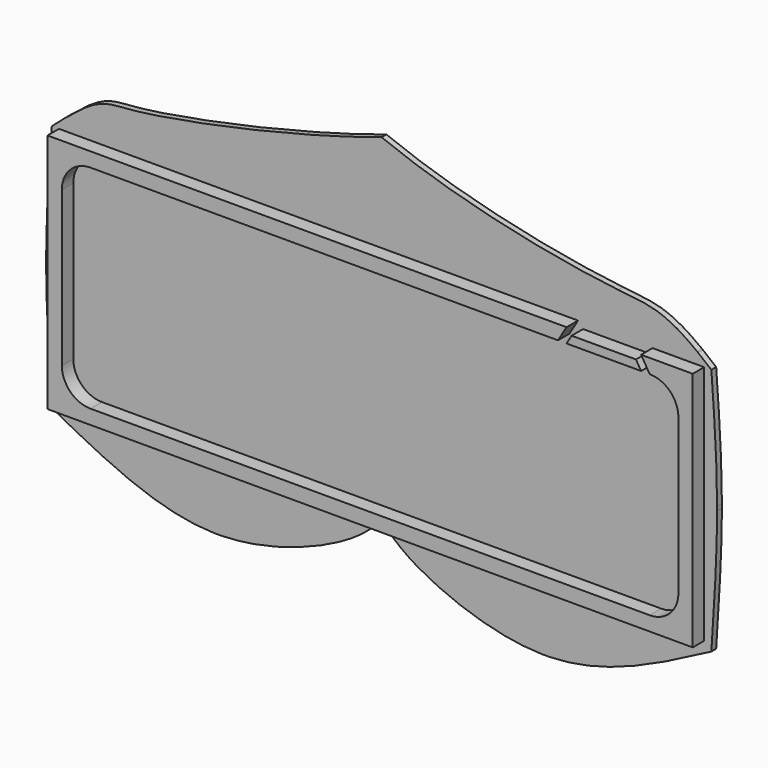
from build123d import *

# Parameters (mm, degrees)
F0_W     = 584.2
F0_H     = 219.71
F1_DEPTH = 5.334
F2_W     = 571.5
F2_H     = 213.36
F2_W_2   = 546.1
F2_H_2   = 187.96
F3_DEPTH = 12.7
F4_R     = 25.4
F6_DEPTH = 12.7
F8_DEPTH = 5.334
F9_DEPTH = 5.334


# Not quite as in the source:
# - a feature names something its author has since deleted; it is built from what else it names


with BuildPart() as f1:
    # F0 (on Front) → F1 (new body)
    with BuildSketch(Plane.XZ):
        with Locations((-292.1, 109.855)):
            Rectangle(F0_W, F0_H)
    extrude(amount=F1_DEPTH)

    # F2 (on face) → F3 (join)
    with BuildSketch(Plane.XZ.offset(5.334)):
        with Locations((-292.1, 113.03)):
            Rectangle(F2_W, F2_H)
        with Locations((-292.1, 113.03)):
            Rectangle(F2_W_2, F2_H_2, mode=Mode.SUBTRACT)
    extrude(amount=F3_DEPTH)

    # F4
    f4_edges = [f1.edges().sort_by_distance(p)[0] for p in [
        (-565.15, -11.684, 207.01),
        (-19.05, -11.684, 207.01),
        (-19.05, -11.684, 19.05),
        (-565.15, -11.684, 19.05),
    ]]
    fillet(f4_edges, radius=F4_R)

    # F5 (on face) → F6 (cut)
    with BuildSketch(Plane.XZ.offset(18.034)):
        Polygon((-118.11, 219.71), (-125.73, 207.01), (-118.11, 207.01), (-113.5820166854, 214.5566388576), (-110.49, 219.71), align=None)
        Polygon((-56.5979833146, 214.5566388576), (-52.07, 207.01), (-44.45, 207.01), (-52.07, 219.71), (-59.69, 219.71), align=None)
        Polygon((-59.69, 219.71), (-110.49, 219.71), (-113.5820166854, 214.5566388576), (-56.5979833146, 214.5566388576), align=None)
    extrude(amount=-F6_DEPTH, mode=Mode.SUBTRACT)

    # F7 (on face) → F8 (cut)
    with BuildSketch(Plane(origin=(0, 0, 0), x_dir=(-1, 0, 0), z_dir=(0, 1, 0))):
        with BuildLine():
            add(Edge.make_bspline(
                [(292.1, 6.35), (289.8878914708, 4.2388101088), (287.6757829415, 2.1276202176), (285.3383261504, 0)],
                knots=[0, 0, 0, 0, 0.0566650496, 0.0566650496, 0.0566650496, 0.0566650496], degree=3))
            Line((285.3383261504, 0), (292.1, 0))
            Line((292.1, 0), (292.1, 6.35))
        make_face()
        with BuildLine():
            add(Edge.make_bspline(
                [(292.1, 6.35), (294.3115112442, 4.2388053382), (296.5230224884, 2.1276106765), (298.8599853109, 0)],
                knots=[0, 0, 0, 0, 0.056662645, 0.056662645, 0.056662645, 0.056662645], degree=3))
            Line((292.1, 6.35), (292.1, 0))
            Line((292.1, 0), (298.8599853109, 0))
        make_face()
    extrude(amount=-F8_DEPTH, mode=Mode.SUBTRACT)

    # F7 (on face) → F9 (join)
    with BuildSketch(Plane(origin=(0, 0, 0), x_dir=(-1, 0, 0), z_dir=(0, 1, 0))):
        with BuildLine():
            Line((285.3383261504, 0), (0, 0))
            add(Edge.make_bspline(
                [(35.5548654074, -18.4164866805), (23.6750755263, -12.5314961521), (11.8375377632, -6.265748076), (0, 0)],
                knots=[0.8952858021, 0.8952858021, 0.8952858021, 0.8952858021, 1, 1, 1, 1], degree=3))
            Line((35.5548654074, -18.4164866805), (260.35, -18.4164866805))
            add(Edge.make_bspline(
                [(285.3383261504, 0), (278.8607301271, -5.8960937002), (271.4205053001, -11.9183662972), (260.35, -18.4164866805)],
                knots=[0.0566650496, 0.0566650496, 0.0566650496, 0.0566650496, 0.2136961022, 0.2136961022, 0.2136961022, 0.2136961022], degree=3))
        make_face()
        with BuildLine():
            add(Edge.make_bspline(
                [(0, 0), (-2.5016001756, 37.5778391816), (-5.0032003512, 75.1556783631), (-5.08, 111.5191693883)],
                knots=[0, 0, 0, 0, 0.4959951232, 0.4959951232, 0.4959951232, 0.4959951232], degree=3))
            Line((0, 0), (0, 219.71))
            add(Edge.make_bspline(
                [(-5.08, 114.935), (-5.0035853497, 150.6697582461), (-2.5017926748, 185.189879123), (0, 219.71)],
                knots=[0.5115421197, 0.5115421197, 0.5115421197, 0.5115421197, 1, 1, 1, 1], degree=3))
            Line((-5.08, 114.935), (-5.08, 111.5191693883))
        make_face()
        with BuildLine():
            Line((260.35, -18.4164866805), (35.5548654074, -18.4164866805))
            add(Edge.make_bspline(
                [(143.5928555626, -50.8), (106.470496214, -50.0055886792), (70.8264502644, -35.8892656507), (35.5548654074, -18.4164866805)],
                knots=[0.5843850409, 0.5843850409, 0.5843850409, 0.5843850409, 0.8952858021, 0.8952858021, 0.8952858021, 0.8952858021], degree=3))
            Line((143.5928555626, -50.8), (150.3785817486, -50.8))
            add(Edge.make_bspline(
                [(260.35, -18.4164866805), (235.5497171967, -32.973656279), (192.5306851802, -49.9188924594), (150.3785817486, -50.8)],
                knots=[0.2136961022, 0.2136961022, 0.2136961022, 0.2136961022, 0.5654790071, 0.5654790071, 0.5654790071, 0.5654790071], degree=3))
        make_face()
        with BuildLine():
            add(Edge.make_bspline(
                [(11.7731056729, 229.2938254471), (8.1151931686, 226.4637173569), (4.2088787391, 223.2851496368), (0, 219.71)],
                knots=[0.9578423111, 0.9578423111, 0.9578423111, 0.9578423111, 1, 1, 1, 1], degree=3))
            Line((0, 219.71), (292.1, 219.71))
            Line((292.1, 219.71), (11.7731056729, 229.2938254471))
        make_face()
        with BuildLine():
            add(Edge.make_bspline(
                [(12.5206463088, 229.87), (12.2726179558, 229.6795636028), (12.0234435309, 229.4875105602), (11.7731056729, 229.2938254471)],
                knots=[0.9549571504, 0.9549571504, 0.9549571504, 0.9549571504, 0.9578423111, 0.9578423111, 0.9578423111, 0.9578423111], degree=3))
            Line((11.7731056729, 229.2938254471), (292.1, 219.71))
            Line((292.1, 219.71), (573.1817260974, 229.3196316614))
            add(Edge.make_bspline(
                [(572.5320605941, 229.87), (572.7473841939, 229.6879525114), (572.9639346328, 229.5045002197), (573.1817260974, 229.3196316614)],
                knots=[0.9616983958, 0.9616983958, 0.9616983958, 0.9616983958, 0.9640299265, 0.9640299265, 0.9640299265, 0.9640299265], degree=3))
            Line((572.5320605941, 229.87), (514.35, 229.87))
            Line((514.35, 229.87), (292.1, 229.87))
            Line((292.1, 229.87), (82.55, 229.87))
            Line((82.55, 229.87), (12.5206463088, 229.87))
        make_face()
        with BuildLine():
            Line((573.1817260974, 229.3196316614), (292.1, 219.71))
            Line((292.1, 219.71), (584.2, 219.71))
            add(Edge.make_bspline(
                [(573.1817260974, 229.3196316614), (576.5417396252, 226.4675416698), (580.1971331881, 223.2783621084), (584.2, 219.71)],
                knots=[0.9640299265, 0.9640299265, 0.9640299265, 0.9640299265, 1, 1, 1, 1], degree=3))
        make_face()
        with BuildLine():
            add(Edge.make_bspline(
                [(298.8599853109, 0), (305.3364495341, -5.8962831133), (312.7764065366, -11.9186444461), (323.85, -18.4164866805)],
                knots=[0.056662645, 0.056662645, 0.056662645, 0.056662645, 0.2136927825, 0.2136927825, 0.2136927825, 0.2136927825], degree=3))
            Line((323.85, -18.4164866805), (548.6673215949, -18.4164866805))
            add(Edge.make_bspline(
                [(548.6673215949, -18.4164866805), (560.540064076, -12.5314899408), (572.370032038, -6.2657449704), (584.2, 0)],
                knots=[0.8952964295, 0.8952964295, 0.8952964295, 0.8952964295, 1, 1, 1, 1], degree=3))
            Line((584.2, 0), (298.8599853109, 0))
        make_face()
        with BuildLine():
            Line((548.6673215949, -18.4164866805), (323.85, -18.4164866805))
            add(Edge.make_bspline(
                [(323.85, -18.4164866805), (348.6543054028, -32.9713340996), (391.6899454814, -49.9118498543), (433.8458201185, -50.8)],
                knots=[0.2136927825, 0.2136927825, 0.2136927825, 0.2136927825, 0.5654325768, 0.5654325768, 0.5654325768, 0.5654325768], degree=3))
            Line((433.8458201185, -50.8), (440.69, -50.8))
            add(Edge.make_bspline(
                [(440.69, -50.8), (477.8051745876, -49.9992725657), (513.4246952416, -35.8853016167), (548.6673215949, -18.4164866805)],
                knots=[0.5844980763, 0.5844980763, 0.5844980763, 0.5844980763, 0.8952964295, 0.8952964295, 0.8952964295, 0.8952964295], degree=3))
        make_face()
        with BuildLine():
            add(Edge.make_bspline(
                [(82.55, 255.27), (55.6261452853, 252.2921647864), (42.3764019315, 252.7932765823), (12.5206463088, 229.87)],
                knots=[0.6076635734, 0.6076635734, 0.6076635734, 0.6076635734, 0.9549571504, 0.9549571504, 0.9549571504, 0.9549571504], degree=3))
            Line((12.5206463088, 229.87), (82.55, 229.87))
            Line((82.55, 229.87), (82.55, 255.27))
        make_face()
        with BuildLine():
            add(Edge.make_bspline(
                [(589.28, 114.935), (589.2035853497, 150.6697582461), (586.7017926748, 185.189879123), (584.2, 219.71)],
                knots=[0.5115421197, 0.5115421197, 0.5115421197, 0.5115421197, 1, 1, 1, 1], degree=3))
            Line((584.2, 219.71), (584.2, 0))
            add(Edge.make_bspline(
                [(584.2, 0), (586.7016001756, 37.5778391816), (589.2032003512, 75.1556783632), (589.28, 111.5191693884)],
                knots=[0, 0, 0, 0, 0.4959951232, 0.4959951232, 0.4959951232, 0.4959951232], degree=3))
            Line((589.28, 111.5191693884), (589.28, 114.935))
        make_face()
        with BuildLine():
            Line((82.55, 255.27), (82.55, 229.87))
            Line((82.55, 229.87), (292.1, 229.87))
            Line((292.1, 229.87), (292.1, 306.07))
            add(Edge.make_bspline(
                [(292.1, 306.07), (218.631118536, 276.3414680958), (129.6589788413, 260.4803525873), (82.55, 255.27)],
                knots=[0, 0, 0, 0, 0.6076635734, 0.6076635734, 0.6076635734, 0.6076635734], degree=3))
        make_face()
        with BuildLine():
            Line((514.35, 229.87), (572.5320605941, 229.87))
            add(Edge.make_bspline(
                [(514.35, 255.27), (536.1096268059, 253.2414037435), (541.9337770664, 255.7396244938), (572.5320605941, 229.87)],
                knots=[0.6303792087, 0.6303792087, 0.6303792087, 0.6303792087, 0.9616983958, 0.9616983958, 0.9616983958, 0.9616983958], degree=3))
            Line((514.35, 255.27), (514.35, 229.87))
        make_face()
        with BuildLine():
            Line((292.1, 306.07), (292.1, 229.87))
            Line((292.1, 229.87), (514.35, 229.87))
            Line((514.35, 229.87), (514.35, 255.27))
            add(Edge.make_bspline(
                [(292.1, 306.07), (373.8620877266, 279.3765068054), (472.9493903602, 259.129676569), (514.35, 255.27)],
                knots=[0, 0, 0, 0, 0.6303792087, 0.6303792087, 0.6303792087, 0.6303792087], degree=3))
        make_face()
    extrude(amount=-F9_DEPTH)


solid = f1.part
